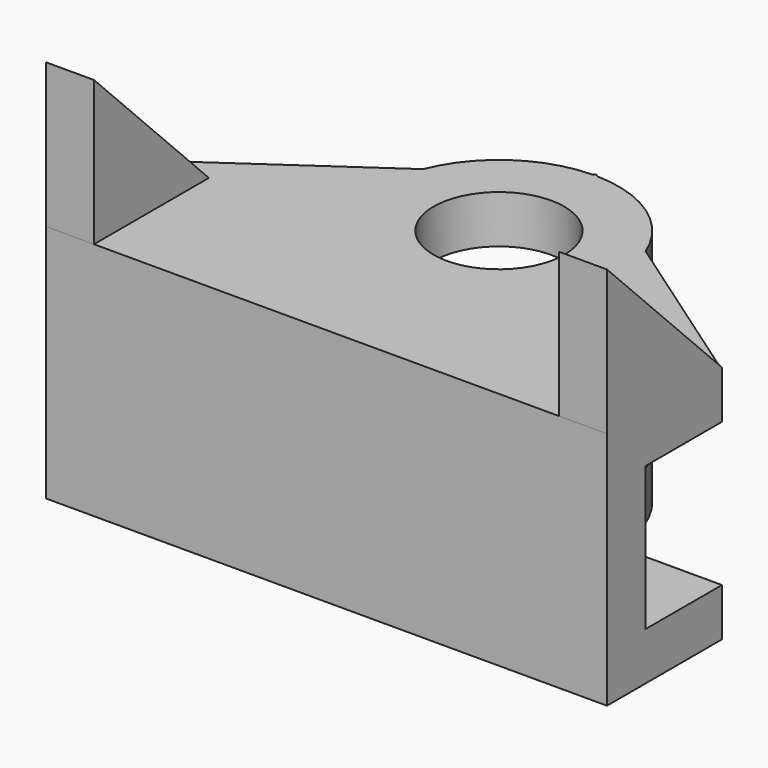
from build123d import *

# Parameters (mm, degrees)
F0_R      = 6.351803
F1_DEPTH  = 6.35
F2_R      = 6.351803
F3_DEPTH  = 3.81
F4_W      = 14.877142
F4_H      = 7.620001
F5_DEPTH  = 6.35
F6_T      = 2.54
F8_DEPTH  = 2.54
F11_START = 3.81
F11_DEPTH = 2.54
F12_R     = 3.466188
F13_DEPTH = 12.7


# Not quite as in the source:
# - a shell that OpenCascade refuses in one call is made with other operations: the cavity is built on its own and cut out


with BuildPart() as f1:
    # F0 (on Top) → F1 (new body, symmetric)
    with BuildSketch(Plane.XY):
        Circle(F0_R)
    extrude(amount=F1_DEPTH, both=True)

    # F2 (on Top) → F3 (cut, symmetric)
    with BuildSketch(Plane.XY):
        Circle(F2_R)
    extrude(amount=F3_DEPTH, both=True, mode=Mode.SUBTRACT)

    # F4 (on Top) → F5 (join, symmetric)
    with BuildSketch(Plane.XY):
        with Locations((-7.438571, -7.62)):
            Rectangle(F4_W, F4_H)
        with Locations((7.438571, -7.62)):
            Rectangle(F4_W, F4_H)
    extrude(amount=F5_DEPTH, both=True)

    # F6: shell of thickness 2.54, made by hand


with BuildPart() as f6_core1:
    # F6_t2: copy of F1
    add(f1.part)

    # the walls: a layer under each face that stays
    f6_faces = [f6_core1.faces().sort_by_distance(p)[0] for p in [
        (0, 6.351803, -5.08),
        (0, 1.270901, -3.81),
        (0, -11.430001, 0),
        (0, 1.270901, 3.81),
        (0, 6.351803, 5.08),
        (0, -2.539099, 6.35),
        (0, -2.539099, -6.35),
    ]]
    thicken(f6_faces, amount=-F6_T, mode=Mode.SUBTRACT)


with BuildPart() as f1_1:
    add(f1.part)

    # what is left inside the walls is the cavity
    f6_cavity = [f6_core1.part.solids().sort_by_distance(p)[0] for p in [
        (0, -3.8354, -1.27),
    ]]
    add(f6_cavity, mode=Mode.SUBTRACT)

    # F7 (on face) → F8 (join)
    with BuildSketch(Plane.YZ.offset(14.877142)):
        Polygon((-11.430001, 14.022371), (-11.430001, 6.35), (-3.81, 6.35), align=None)
    extrude(amount=-F8_DEPTH)

    # F9: F1 across plane


with BuildPart() as f1_2:
    add(f1_1.part)
    add(f1_1.part.mirror(Plane.YZ))

    # F10 (on Top) → F11 (join)
    with BuildSketch(Plane.XY.offset(F11_START)):
        Polygon((0, -3.819642), (0, 6.448444), (-14.77987, -3.819642), align=None)
        Polygon((14.77987, -3.819642), (0, 6.448444), (0, -3.819642), align=None)
    extrude(amount=F11_DEPTH)

    # F12 (on Top) → F13 (cut, symmetric)
    with BuildSketch(Plane.XY):
        Circle(F12_R)
    extrude(amount=F13_DEPTH, both=True, mode=Mode.SUBTRACT)


solid = f1_2.part
